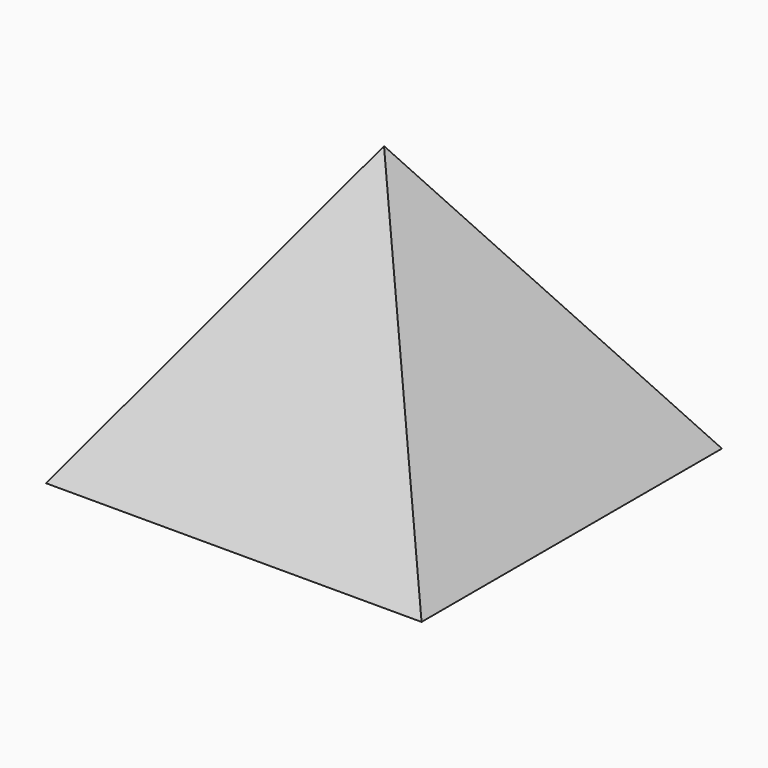
from build123d import *

# Parameters (mm, degrees)
F0_W     = 40
F0_H     = 40
F1_DEPTH = 30
F2_SIZE2 = 29.99999
F2_SIZE  = 19.99999


# Not quite as in the source:
# - a fillet or chamfer is up to 0.001 mm smaller than in the source, because OpenCascade refuses the exact size


with BuildPart() as f1:
    # F0 (on Top) → F1 (new body)
    with BuildSketch(Plane.XY):
        Rectangle(F0_W, F0_H)
    extrude(amount=F1_DEPTH)

    # F2 (size 20 and 30 in the source; OpenCascade refuses exactly that, so slightly less here)
    f2_edges = [f1.edges().sort_by_distance(p)[0] for p in [
        (-20, 0, 30),
        (0, 20, 30),
        (0, -20, 30),
        (20, 0, 30),
    ]]
    f2_side = f1.faces().sort_by_distance((0, 0, 30))[0]
    chamfer(f2_edges, length=F2_SIZE, length2=F2_SIZE2, reference=f2_side)


solid = f1.part
